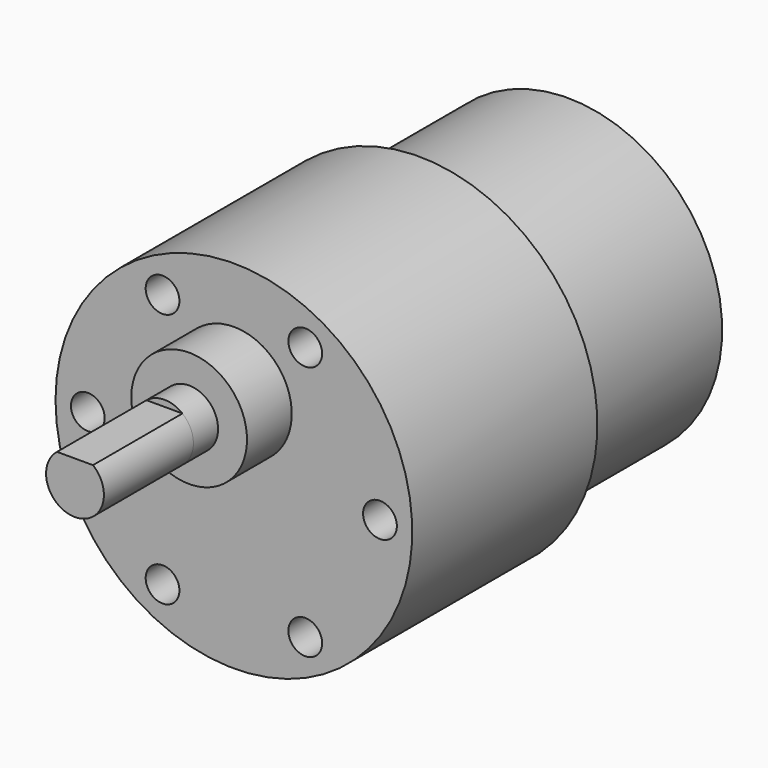
from build123d import *

# Parameters (mm, degrees)
F1_DEPTH  = 11.6
F3_R      = 3
F4_DEPTH  = 3.2
F6_R      = 6
F7_DEPTH  = 5.8
F9_R      = 18.5
F10_DEPTH = 24
F12_R     = 16
F13_DEPTH = 19.3
F14_R     = 1.75
F15_DEPTH = 4


# Not quite as in the source:
# - after a boolean that leaves OpenCascade's solid faulty, fix() repairs it


with BuildPart() as f1:
    # F0 (on Front) → F1 (new body)
    with BuildSketch(Plane.XZ):
        with BuildLine():
            Line((1.8648056199, 2.35), (-1.8648056199, 2.35))
            ThreePointArc((-1.8648056199, 2.35), (0, -3), (1.8648056199, 2.35))
        make_face()
    extrude(amount=-F1_DEPTH)

    # F3 (on offset) → F4 (join)
    with BuildSketch(Plane(origin=(0, 11.6, 0), x_dir=(-1, 0, 0), z_dir=(0, 1, 0))):
        Circle(F3_R)
    extrude(amount=F4_DEPTH)

    # F6 (on offset) → F7 (join)
    with BuildSketch(Plane(origin=(0, 14.8, 0), x_dir=(-1, 0, 0), z_dir=(0, 1, 0))):
        Circle(F6_R)
    extrude(amount=F7_DEPTH)

    add(f1.part.fix(), mode=Mode.REPLACE)

    # F9 (on offset) → F10 (join)
    with BuildSketch(Plane(origin=(0, 20.6, 0), x_dir=(-1, 0, 0), z_dir=(0, 1, 0))):
        with Locations((0, -6.7)):
            Circle(F9_R)
    extrude(amount=F10_DEPTH)

    # F12 (on offset) → F13 (join)
    with BuildSketch(Plane(origin=(0, 44.6, 0), x_dir=(-1, 0, 0), z_dir=(0, 1, 0))):
        with Locations((0, -6.7)):
            Circle(F12_R)
    extrude(amount=F13_DEPTH)

    # F14 (on offset) → F15 (cut)
    with BuildSketch(Plane(origin=(0, 20.6, 0), x_dir=(-1, 0, 0), z_dir=(0, 1, 0))):
        with Locations((-15.15, -6.7)):
            Circle(F14_R)
        with Locations((15.15, -6.7)):
            Circle(F14_R)
        with Locations((7.4, -19.9197768514)):
            Circle(F14_R)
        with Locations((-7.4, -19.9197768514)):
            Circle(F14_R)
        with Locations((-7.4, 6.5197768514)):
            Circle(F14_R)
        with Locations((7.4, 6.5197768514)):
            Circle(F14_R)
    extrude(amount=F15_DEPTH, mode=Mode.SUBTRACT)


solid = f1.part
